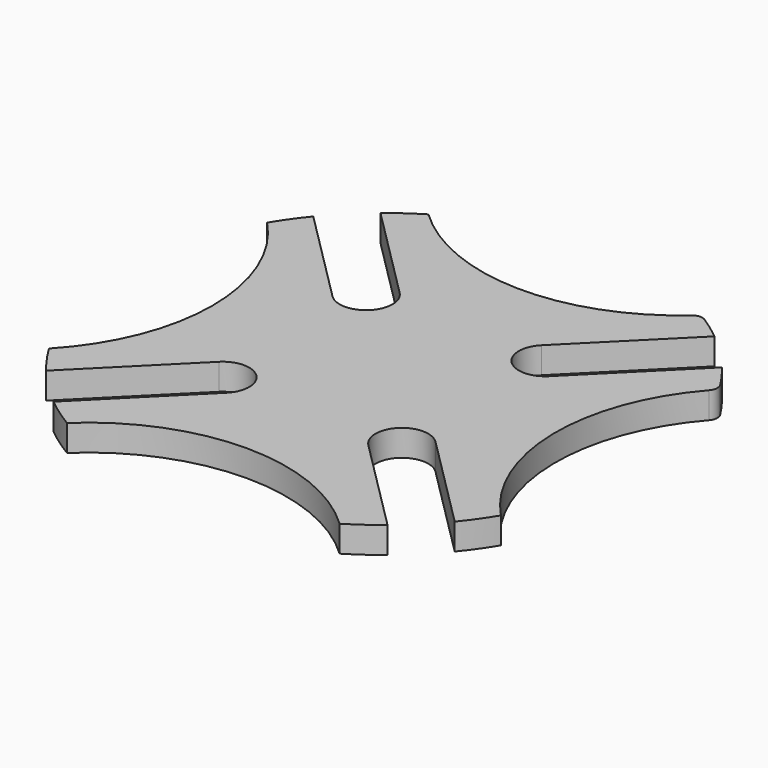
from build123d import *

# Parameters (mm, degrees)
F1_DEPTH = 12.7
F3_R     = 5.08
F4_DEPTH = 25.4


with BuildPart() as f1:
    # F0 (on Top) → F1 (new body)
    with BuildSketch(Plane.XY):
        with BuildLine():
            ThreePointArc((108.74375, -65.6033294577), (82.55, 0), (108.74375, 65.6033294577))
            ThreePointArc((108.74375, 65.6033294577), (89.8025612107, 89.8025612107), (65.6033294577, 108.74375))
            ThreePointArc((65.6033294577, 108.74375), (0, 82.55), (-65.6033294577, 108.74375))
            ThreePointArc((-65.6033294577, 108.74375), (-89.8025612107, 89.8025612107), (-108.74375, 65.6033294577))
            ThreePointArc((-108.74375, 65.6033294577), (-82.55, 0), (-108.74375, -65.6033294577))
            ThreePointArc((-108.74375, -65.6033294577), (-89.8025612107, -89.8025612107), (-65.6033294577, -108.74375))
            ThreePointArc((-65.6033294577, -108.74375), (0, -82.55), (65.6033294577, -108.74375))
            ThreePointArc((65.6033294577, -108.74375), (89.8025612107, -89.8025612107), (108.74375, -65.6033294577))
        make_face()
    extrude(amount=F1_DEPTH)

    # F3
    f3_edges = [f1.edges().sort_by_distance(p)[0] for p in [
        (65.603329, 108.74375, 6.35),
        (108.74375, 65.603329, 6.35),
    ]]
    fillet(f3_edges, radius=F3_R)

    # F2 (on face) → F4 (cut)
    with BuildSketch(Plane.XY.offset(12.7)):
        with BuildLine():
            Line((105.9670222286, 88.0065099865), (96.9867661075, 96.9867661075))
            Line((96.9867661075, 96.9867661075), (88.0065099865, 105.9670222286))
            Line((88.0065099865, 105.9670222286), (34.1249732601, 52.0854855022))
            ThreePointArc((34.1249732601, 52.0854855022), (34.1249732601, 34.1249732601), (52.0854855022, 34.1249732601))
            Line((52.0854855022, 34.1249732601), (105.9670222286, 88.0065099865))
        make_face()
        with BuildLine():
            ThreePointArc((-52.0854855022, 34.1249732601), (-34.1249732601, 34.1249732601), (-34.1249732601, 52.0854855022))
            Line((-34.1249732601, 52.0854855022), (-88.0065099865, 105.9670222286))
            Line((-88.0065099865, 105.9670222286), (-96.9867661075, 96.9867661075))
            Line((-96.9867661075, 96.9867661075), (-105.9670222286, 88.0065099865))
            Line((-105.9670222286, 88.0065099865), (-52.0854855022, 34.1249732601))
        make_face()
        with BuildLine():
            Line((-88.0065099865, -105.9670222286), (-34.1249732601, -52.0854855022))
            ThreePointArc((-34.1249732601, -52.0854855022), (-34.1249732601, -34.1249732601), (-52.0854855022, -34.1249732601))
            Line((-52.0854855022, -34.1249732601), (-105.9670222286, -88.0065099865))
            Line((-105.9670222286, -88.0065099865), (-96.9867661075, -96.9867661075))
            Line((-96.9867661075, -96.9867661075), (-88.0065099865, -105.9670222286))
        make_face()
        with BuildLine():
            Line((34.1249732601, -52.0854855022), (88.0065099865, -105.9670222286))
            Line((88.0065099865, -105.9670222286), (96.9867661075, -96.9867661075))
            Line((96.9867661075, -96.9867661075), (105.9670222286, -88.0065099865))
            Line((105.9670222286, -88.0065099865), (52.0854855022, -34.1249732601))
            ThreePointArc((52.0854855022, -34.1249732601), (34.1249732601, -34.1249732601), (34.1249732601, -52.0854855022))
        make_face()
    extrude(amount=-F4_DEPTH, mode=Mode.SUBTRACT)


solid = f1.part
